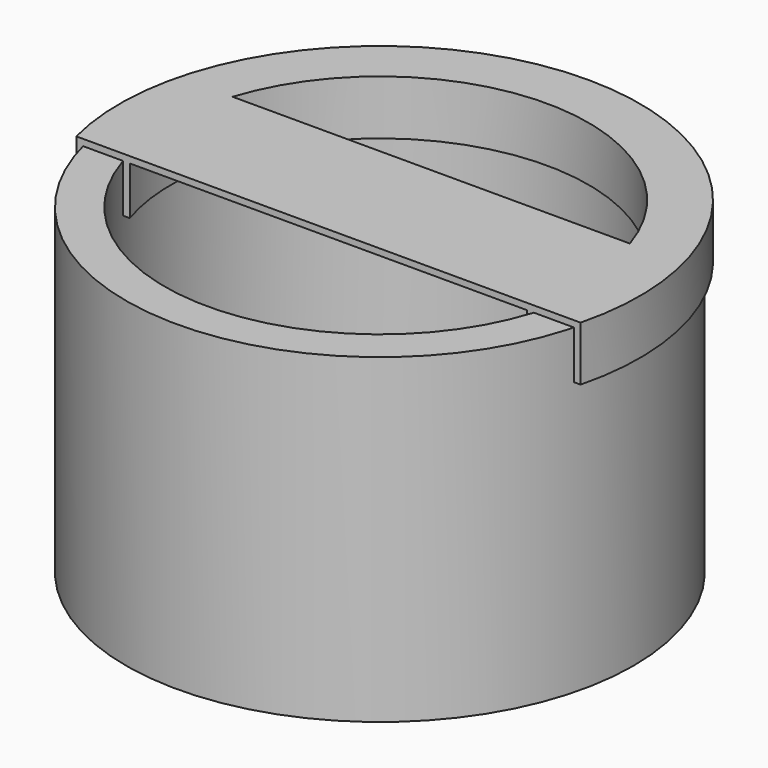
from build123d import *

# Parameters (mm, degrees)
F0_R        = 79
F0_R_2      = 67
F1_DEPTH    = 100
F2_R        = 81
F2_R_2      = 79
F3_DEPTH    = 15
F2_R_3      = 67
F1_FACE_R   = 79
F1_FACE_R_2 = 67
F4_DEPTH    = 2
F6_DEPTH    = 25


with BuildPart() as f1:
    # F0 (on Top) → F1 (new body)
    with BuildSketch(Plane.XY):
        Circle(F0_R)
        Circle(F0_R_2, mode=Mode.SUBTRACT)
    extrude(amount=F1_DEPTH)


with BuildPart() as f3:
    # F2 (on face) → F3 (new body)
    with BuildSketch(Plane.XY.offset(100)):
        Circle(F2_R)
        Circle(F2_R_2, mode=Mode.SUBTRACT)
    extrude(amount=-F3_DEPTH)



with BuildPart() as f3b:
    # F2 (on face) → F3, piece 2 (new body)
    with BuildSketch(Plane.XY.offset(100)):
        Circle(F2_R_3)
        with BuildLine():
            ThreePointArc((61.8465843843, 20), (64.2068064343, 10.1235373023), (65, 0))
            ThreePointArc((65, 0), (64.2068064343, -10.1235373023), (61.8465843843, -20))
            ThreePointArc((61.8465843843, -20), (0, -65), (-61.8465843843, -20))
            ThreePointArc((-61.8465843843, -20), (-65, 0), (-61.8465843843, 20))
            ThreePointArc((-61.8465843843, 20), (0, 65), (61.8465843843, 20))
        make_face(mode=Mode.SUBTRACT)
    extrude(amount=-F3_DEPTH)


with BuildPart() as f3_1:
    add(f3.part)

    add(f3b.part)  # F4 merges F3b
    # F2 (on face) + F1_face (on face) → F4 (join)
    with BuildSketch(Plane.XY.offset(100)):
        Circle(F2_R)
        Circle(F2_R_2, mode=Mode.SUBTRACT)
        Circle(F2_R_3)
        with BuildLine():
            ThreePointArc((61.8465843843, 20), (64.2068064343, 10.1235373023), (65, 0))
            ThreePointArc((65, 0), (64.2068064343, -10.1235373023), (61.8465843843, -20))
            ThreePointArc((61.8465843843, -20), (0, -65), (-61.8465843843, -20))
            ThreePointArc((-61.8465843843, -20), (-65, 0), (-61.8465843843, 20))
            ThreePointArc((-61.8465843843, 20), (0, 65), (61.8465843843, 20))
        make_face(mode=Mode.SUBTRACT)
        with BuildLine():
            ThreePointArc((61.8465843843, -20), (64.2068064343, -10.1235373023), (65, 0))
            ThreePointArc((65, 0), (64.2068064343, 10.1235373023), (61.8465843843, 20))
            Line((61.8465843843, 20), (-61.8465843843, 20))
            ThreePointArc((-61.8465843843, 20), (-65, 0), (-61.8465843843, -20))
            Line((-61.8465843843, -20), (61.8465843843, -20))
        make_face()
    with BuildSketch(Plane.XY.offset(100)):
        Circle(F1_FACE_R)
        Circle(F1_FACE_R_2, mode=Mode.SUBTRACT)
    extrude(amount=F4_DEPTH)

    # F5 (on face) → F6 (cut)
    with BuildSketch(Plane.XY.offset(102)):
        Polygon((109.0431064367, -96.566259861), (109.0431064367, -20), (61.8465843843, -20), (-61.8465843843, -20), (-82.0130482316, -20), (-82.0130482316, -96.566259861), align=None)
    extrude(amount=-F6_DEPTH, mode=Mode.SUBTRACT)


solid = Compound([f1.part, f3_1.part])
